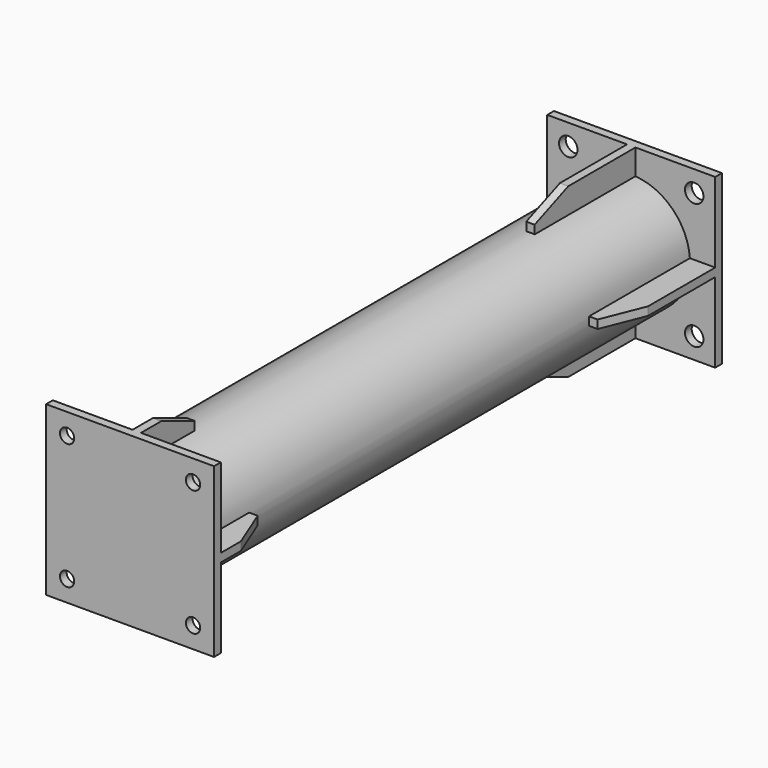
from build123d import *

# Parameters (mm, degrees)
F0_R          = 70
F0_R_2        = 65
F1_DEPTH      = 736
F2_W          = 200
F2_H          = 200
F2_R          = 11
F3_DEPTH      = 10
F4_W          = 30.1787997812
F4_H          = 10
F4_W_2        = 10
F4_H_2        = 30.1787997812
F5_DEPTH      = 150
F6_T1_DEPTH   = 269.311363913
F6_T3_DEPTH   = 269.311363913
F6_T8_DEPTH   = 269.311363913
F6_S9_R       = 70
F6_T10_DEPTH  = 139
F8_W          = 200
F8_H          = 200
F8_R          = 8.5
F9_DEPTH      = 10
F10_W         = 10
F10_H         = 30.1787997812
F10_W_2       = 30.1787997812
F10_H_2       = 10
F11_DEPTH     = 80
F12_T1_DEPTH  = 269.311363913
F12_T3_DEPTH  = 269.311363913
F12_T8_DEPTH  = 269.311363913
F12_S9_R      = 70
F12_T10_DEPTH = 139
F12_T14_DEPTH = 269.311363913
F12_S15_R     = 70
F12_T16_DEPTH = 139


# Not quite as in the source:
# - a fillet or chamfer that OpenCascade refuses, or shapes differently, is made with other operations: its cross-section is extruded or revolved along the edge and cut away or added


with BuildPart() as f1:
    # F0 (on Front) → F1 (new body)
    with BuildSketch(Plane.XZ):
        Circle(F0_R)
        Circle(F0_R_2, mode=Mode.SUBTRACT)
    extrude(amount=F1_DEPTH)

    # F2 (on Front) → F3 (join)
    with BuildSketch(Plane.XZ):
        Rectangle(F2_W, F2_H)
        with Locations((-75, -75)):
            Circle(F2_R, mode=Mode.SUBTRACT)
        with Locations((75, -75)):
            Circle(F2_R, mode=Mode.SUBTRACT)
        with Locations((-75, 75)):
            Circle(F2_R, mode=Mode.SUBTRACT)
        with Locations((75, 75)):
            Circle(F2_R, mode=Mode.SUBTRACT)
    extrude(amount=-F3_DEPTH)

    # F4 (on Front) → F5 (join)
    with BuildSketch(Plane.XZ):
        with Locations((-84.9106001094, 0)):
            Rectangle(F4_W, F4_H)
        with Locations((0, 84.9106001094)):
            Rectangle(F4_W_2, F4_H_2)
        with Locations((84.9106001094, 0)):
            Rectangle(F4_W, F4_H)
        with Locations((0, -84.9106001094)):
            Rectangle(F4_W_2, F4_H_2)
    extrude(amount=F5_DEPTH)

    # F6: chamfer of 50 x 20 on 4 edges, made by hand

    # F6_s2 → F6_t1 (cut)
    with BuildSketch(Plane.YZ.offset(-134.6556819565)):
        Polygon((-100, 100), (-150, 80), (-150, 100), align=None)
        Polygon((-100, -100), (-150, -80), (-150, -100), align=None)
    extrude(amount=F6_T1_DEPTH, mode=Mode.SUBTRACT)

    # F6_s4 → F6_t3 (cut)
    with BuildSketch(Plane.XY.offset(-134.6556819565)):
        Polygon((100, -100), (80, -150), (100, -150), align=None)
    extrude(amount=F6_T3_DEPTH, mode=Mode.SUBTRACT)


with BuildPart() as f6_tool6:
    # F6_s7 → F6_t8 (new body)
    with BuildSketch(Plane.XY.offset(134.6556819565)):
        Polygon((-100, -130), (-50, -150), (-100, -150), align=None)
    extrude(amount=-F6_T8_DEPTH)

    # F6_s9 → F6_t10 (cut, symmetric)
    with BuildSketch(Plane.XZ.offset(140)):
        Circle(F6_S9_R)
    extrude(amount=F6_T10_DEPTH, both=True, mode=Mode.SUBTRACT)


with BuildPart() as f1_1:
    add(f1.part)

    # F6_t5: cut F6_tool6
    add(f6_tool6.part, mode=Mode.SUBTRACT)

    # F8 (on offset) → F9 (join)
    with BuildSketch(Plane.XZ.offset(736)):
        Rectangle(F8_W, F8_H)
        with Locations((-75, -75)):
            Circle(F8_R, mode=Mode.SUBTRACT)
        with Locations((75, -75)):
            Circle(F8_R, mode=Mode.SUBTRACT)
        with Locations((-75, 75)):
            Circle(F8_R, mode=Mode.SUBTRACT)
        with Locations((75, 75)):
            Circle(F8_R, mode=Mode.SUBTRACT)
    extrude(amount=F9_DEPTH)

    # F10 (on face) → F11 (join)
    with BuildSketch(Plane(origin=(0, -736, 0), x_dir=(-1, 0, 0), z_dir=(0, 1, 0))):
        with Locations((0, 84.9106001094)):
            Rectangle(F10_W, F10_H)
        with Locations((84.9106001094, 0)):
            Rectangle(F10_W_2, F10_H_2)
        with Locations((0, -84.9106001094)):
            Rectangle(F10_W, F10_H)
        with Locations((-84.9106001094, 0)):
            Rectangle(F10_W_2, F10_H_2)
    extrude(amount=F11_DEPTH)

    # F12: chamfer of 20 x 50 on 4 edges, made by hand

    # F12_s2 → F12_t1 (cut)
    with BuildSketch(Plane.YZ.offset(-134.6556819565)):
        Polygon((-706, 100), (-656, 80), (-656, 100), align=None)
    extrude(amount=F12_T1_DEPTH, mode=Mode.SUBTRACT)

    # F12_s4 → F12_t3 (cut)
    with BuildSketch(Plane.XY.offset(-134.6556819565)):
        Polygon((100, -706), (80, -656), (100, -656), align=None)
    extrude(amount=F12_T3_DEPTH, mode=Mode.SUBTRACT)


with BuildPart() as f12_tool6:
    # F12_s7 → F12_t8 (new body)
    with BuildSketch(Plane.XY.offset(-134.6556819565)):
        Polygon((-100, -676), (-50, -656), (-100, -656), align=None)
    extrude(amount=F12_T8_DEPTH)

    # F12_s9 → F12_t10 (cut, symmetric)
    with BuildSketch(Plane.XZ.offset(666)):
        Circle(F12_S9_R)
    extrude(amount=F12_T10_DEPTH, both=True, mode=Mode.SUBTRACT)


with BuildPart() as f1_2:
    add(f1_1.part)

    # F12_t5: cut F12_tool6
    add(f12_tool6.part, mode=Mode.SUBTRACT)


with BuildPart() as f12_tool12:
    # F12_s13 → F12_t14 (new body)
    with BuildSketch(Plane.YZ.offset(134.6556819565)):
        Polygon((-676, -100), (-656, -50), (-656, -100), align=None)
    extrude(amount=-F12_T14_DEPTH)

    # F12_s15 → F12_t16 (cut, symmetric)
    with BuildSketch(Plane.XZ.offset(666)):
        Circle(F12_S15_R)
    extrude(amount=F12_T16_DEPTH, both=True, mode=Mode.SUBTRACT)


with BuildPart() as f1_3:
    add(f1_2.part)

    # F12_t11: cut F12_tool12
    add(f12_tool12.part, mode=Mode.SUBTRACT)


solid = f1_3.part
